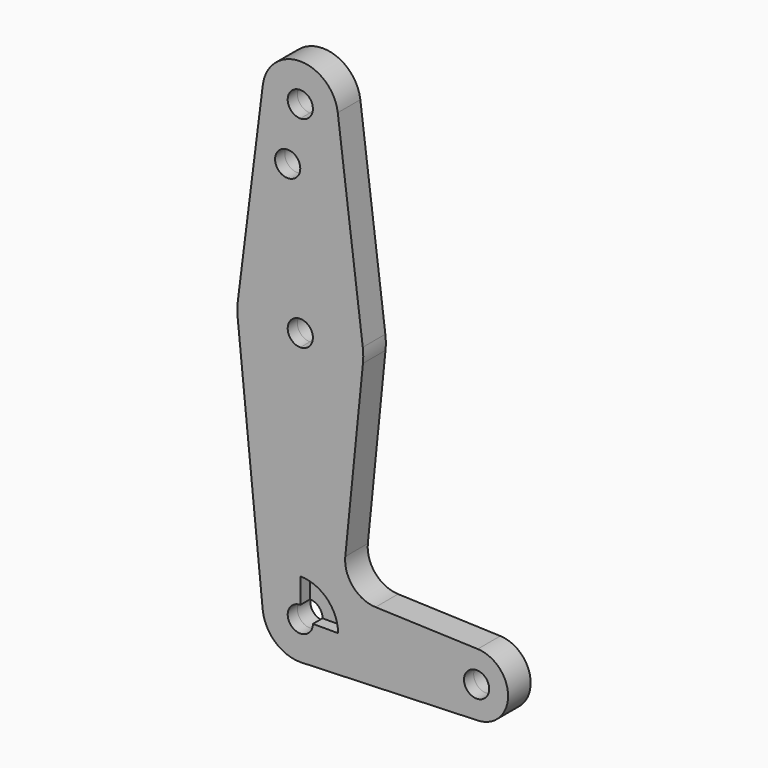
from build123d import *

# Parameters (mm, degrees)
F0_R     = 3.175
F1_DEPTH = 4.064
F2_DEPTH = 3.048


with BuildPart() as f1:
    # F0 (on Front) → F1 (new body)
    with BuildSketch(Plane.XZ):
        with BuildLine():
            ThreePointArc((15.7954255641, -1.5875), (15.8550939106, -0.7947465541), (15.875, 0))
            ThreePointArc((15.875, 0), (15.8438414904, 0.9941387366), (15.7504882737, 1.984375))
            ThreePointArc((15.7504882737, 1.984375), (10.5003255158, 11.90625), (0, 15.875))
            Line((0, 15.875), (0, 3.175))
            ThreePointArc((0, 3.175), (2.2450640303, 2.2450640303), (3.175, 0))
            ThreePointArc((3.175, 0), (2.2450640303, -2.2450640303), (0, -3.175))
            Line((0, -3.175), (0, -15.875))
            ThreePointArc((0, -15.875), (10.6492737428, -11.7732150983), (15.7954255641, -1.5875))
        make_face()
        with BuildLine():
            ThreePointArc((0, 15.875), (10.5003255158, 11.90625), (15.7504882737, 1.984375))
            Line((15.7504882737, 1.984375), (9.4502929642, 51.990625))
            ThreePointArc((9.4502929642, 51.990625), (9.5063048942, 51.396483242), (9.525, 50.8))
            ThreePointArc((9.525, 50.8), (6.7351920908, 44.0648079092), (0, 41.275))
            Line((0, 41.275), (0, 36.5252))
            Line((0, 36.5252), (0, 29.7381002456))
            Line((0, 29.7381002456), (0, 15.875))
        make_face()
        with BuildLine():
            Line((11.3411865923, -45.9066181876), (15.7954255641, -1.5875))
            ThreePointArc((15.7954255641, -1.5875), (10.6492737428, -11.7732150983), (0, -15.875))
            Line((0, -15.875), (0, -53.975))
            ThreePointArc((0, -53.975), (6.7351920908, -56.7648079092), (9.525, -63.5))
            Line((9.525, -63.5), (36.5125, -63.5))
            ThreePointArc((36.5125, -63.5), (38.9384772185, -57.7879930953), (44.7334821429, -55.5675637964))
            Line((44.7334821429, -55.5675637964), (18.9676000005, -54.6467662892))
            ThreePointArc((18.9676000005, -54.6467662892), (13.2611998974, -51.9286408502), (11.3411865923, -45.9066181876))
        make_face()
        with BuildLine():
            Line((0, 3.175), (0, 15.875))
            ThreePointArc((0, 15.875), (-10.5003255158, 11.90625), (-15.7504882737, 1.984375))
            ThreePointArc((-15.7504882737, 1.984375), (-15.8737438155, 0.1997054867), (-15.7954255641, -1.5875))
            ThreePointArc((-15.7954255641, -1.5875), (-10.6492737428, -11.7732150983), (0, -15.875))
            Line((0, -15.875), (0, -3.175))
            ThreePointArc((0, -3.175), (-3.175, 0), (0, 3.175))
        make_face()
        with BuildLine():
            ThreePointArc((-15.7504882737, 1.984375), (-10.5003255158, 11.90625), (0, 15.875))
            Line((0, 15.875), (0, 29.7381002456))
            Line((0, 29.7381002456), (0, 36.5252))
            Line((0, 36.5252), (0, 41.275))
            ThreePointArc((0, 41.275), (-7.14375, 44.4998046905), (-9.4502929642, 51.990625))
            Line((-9.4502929642, 51.990625), (-15.7504882737, 1.984375))
        make_face()
        with Locations((-3.175, 36.5252)):
            Circle(F0_R, mode=Mode.SUBTRACT)
        with BuildLine():
            ThreePointArc((9.525, 50.8), (9.5063048942, 51.396483242), (9.4502929642, 51.990625))
            ThreePointArc((9.4502929642, 51.990625), (0, 60.325), (-9.4502929642, 51.990625))
            ThreePointArc((-9.4502929642, 51.990625), (-7.14375, 44.4998046905), (0, 41.275))
            ThreePointArc((0, 41.275), (6.7351920908, 44.0648079092), (9.525, 50.8))
        make_face()
        with BuildLine():
            ThreePointArc((3.175, 50.8), (2.2450640303, 48.5549359697), (0, 47.625))
            ThreePointArc((0, 47.625), (-2.2450640303, 53.0450640303), (3.175, 50.8))
        make_face(mode=Mode.SUBTRACT)
        with BuildLine():
            Line((0, -53.975), (0, -15.875))
            ThreePointArc((0, -15.875), (-10.6492737428, -11.7732150983), (-15.7954255641, -1.5875))
            Line((-15.7954255641, -1.5875), (-9.4772553384, -64.4525))
            ThreePointArc((-9.4772553384, -64.4525), (-7.063929059, -57.1104357543), (0, -53.975))
        make_face()
        with BuildLine():
            Line((0, -60.325), (0, -53.975))
            ThreePointArc((0, -53.975), (-7.063929059, -57.1104357543), (-9.4772553384, -64.4525))
            ThreePointArc((-9.4772553384, -64.4525), (-6.3895642457, -70.563929059), (0, -73.025))
            Line((0, -73.025), (0.6773435479, -73.000885786))
            ThreePointArc((0.6773435479, -73.000885786), (6.9705567315, -69.9912990883), (9.525, -63.5))
            Line((9.525, -63.5), (3.175, -63.5))
            ThreePointArc((3.175, -63.5), (-2.2450640303, -65.7450640303), (0, -60.325))
        make_face()
        with BuildLine():
            Line((36.5125, -63.5), (9.525, -63.5))
            ThreePointArc((9.525, -63.5), (6.9705567315, -69.9912990883), (0.6773435479, -73.000885786))
            Line((0.6773435479, -73.000885786), (44.7324052746, -71.4324746146))
            ThreePointArc((44.7324052746, -71.4324746146), (38.9380895153, -69.2116327839), (36.5125, -63.5))
        make_face()
        with BuildLine():
            ThreePointArc((52.3875, -63.5), (50.1620069047, -57.9884772185), (44.7334821429, -55.5675637964))
            ThreePointArc((44.7334821429, -55.5675637964), (38.9384772185, -57.7879930953), (36.5125, -63.5))
            ThreePointArc((36.5125, -63.5), (38.9380895153, -69.2116327839), (44.7324052746, -71.4324746146))
            ThreePointArc((44.7324052746, -71.4324746146), (50.1616327839, -69.0119104847), (52.3875, -63.5))
        make_face()
        with BuildLine():
            ThreePointArc((47.625, -63.5), (44.45, -66.675), (41.275, -63.5))
            ThreePointArc((41.275, -63.5), (44.45, -60.325), (47.625, -63.5))
        make_face(mode=Mode.SUBTRACT)
        with BuildLine():
            Line((0.6773435479, -73.000885786), (0, -73.025))
            ThreePointArc((0, -73.025), (0.3388863295, -73.0189695375), (0.6773435479, -73.000885786))
        make_face()
        with BuildLine():
            ThreePointArc((9.525, -63.5), (6.7351920908, -56.7648079092), (0, -53.975))
            Line((0, -53.975), (0, -60.325))
            ThreePointArc((0, -60.325), (2.2450640303, -61.2549359697), (3.175, -63.5))
            Line((3.175, -63.5), (9.525, -63.5))
        make_face()
    extrude(amount=-F1_DEPTH)

    # F0 (on Front) → F2 (join)
    with BuildSketch(Plane.XZ):
        with BuildLine():
            ThreePointArc((15.7954255641, -1.5875), (15.8550939106, -0.7947465541), (15.875, 0))
            ThreePointArc((15.875, 0), (15.8438414904, 0.9941387366), (15.7504882737, 1.984375))
            ThreePointArc((15.7504882737, 1.984375), (10.5003255158, 11.90625), (0, 15.875))
            Line((0, 15.875), (0, 3.175))
            ThreePointArc((0, 3.175), (2.2450640303, 2.2450640303), (3.175, 0))
            ThreePointArc((3.175, 0), (2.2450640303, -2.2450640303), (0, -3.175))
            Line((0, -3.175), (0, -15.875))
            ThreePointArc((0, -15.875), (10.6492737428, -11.7732150983), (15.7954255641, -1.5875))
        make_face()
        with BuildLine():
            ThreePointArc((0, 15.875), (10.5003255158, 11.90625), (15.7504882737, 1.984375))
            Line((15.7504882737, 1.984375), (9.4502929642, 51.990625))
            ThreePointArc((9.4502929642, 51.990625), (9.5063048942, 51.396483242), (9.525, 50.8))
            ThreePointArc((9.525, 50.8), (6.7351920908, 44.0648079092), (0, 41.275))
            Line((0, 41.275), (0, 36.5252))
            Line((0, 36.5252), (0, 29.7381002456))
            Line((0, 29.7381002456), (0, 15.875))
        make_face()
        with BuildLine():
            Line((11.3411865923, -45.9066181876), (15.7954255641, -1.5875))
            ThreePointArc((15.7954255641, -1.5875), (10.6492737428, -11.7732150983), (0, -15.875))
            Line((0, -15.875), (0, -53.975))
            ThreePointArc((0, -53.975), (6.7351920908, -56.7648079092), (9.525, -63.5))
            Line((9.525, -63.5), (36.5125, -63.5))
            ThreePointArc((36.5125, -63.5), (38.9384772185, -57.7879930953), (44.7334821429, -55.5675637964))
            Line((44.7334821429, -55.5675637964), (18.9676000005, -54.6467662892))
            ThreePointArc((18.9676000005, -54.6467662892), (13.2611998974, -51.9286408502), (11.3411865923, -45.9066181876))
        make_face()
        with BuildLine():
            Line((0, 3.175), (0, 15.875))
            ThreePointArc((0, 15.875), (-10.5003255158, 11.90625), (-15.7504882737, 1.984375))
            ThreePointArc((-15.7504882737, 1.984375), (-15.8737438155, 0.1997054867), (-15.7954255641, -1.5875))
            ThreePointArc((-15.7954255641, -1.5875), (-10.6492737428, -11.7732150983), (0, -15.875))
            Line((0, -15.875), (0, -3.175))
            ThreePointArc((0, -3.175), (-3.175, 0), (0, 3.175))
        make_face()
        with BuildLine():
            ThreePointArc((-15.7504882737, 1.984375), (-10.5003255158, 11.90625), (0, 15.875))
            Line((0, 15.875), (0, 29.7381002456))
            Line((0, 29.7381002456), (0, 36.5252))
            Line((0, 36.5252), (0, 41.275))
            ThreePointArc((0, 41.275), (-7.14375, 44.4998046905), (-9.4502929642, 51.990625))
            Line((-9.4502929642, 51.990625), (-15.7504882737, 1.984375))
        make_face()
        with Locations((-3.175, 36.5252)):
            Circle(F0_R, mode=Mode.SUBTRACT)
        with BuildLine():
            ThreePointArc((9.525, 50.8), (9.5063048942, 51.396483242), (9.4502929642, 51.990625))
            ThreePointArc((9.4502929642, 51.990625), (0, 60.325), (-9.4502929642, 51.990625))
            ThreePointArc((-9.4502929642, 51.990625), (-7.14375, 44.4998046905), (0, 41.275))
            ThreePointArc((0, 41.275), (6.7351920908, 44.0648079092), (9.525, 50.8))
        make_face()
        with BuildLine():
            ThreePointArc((3.175, 50.8), (2.2450640303, 48.5549359697), (0, 47.625))
            ThreePointArc((0, 47.625), (-2.2450640303, 53.0450640303), (3.175, 50.8))
        make_face(mode=Mode.SUBTRACT)
        with BuildLine():
            Line((0, -53.975), (0, -15.875))
            ThreePointArc((0, -15.875), (-10.6492737428, -11.7732150983), (-15.7954255641, -1.5875))
            Line((-15.7954255641, -1.5875), (-9.4772553384, -64.4525))
            ThreePointArc((-9.4772553384, -64.4525), (-7.063929059, -57.1104357543), (0, -53.975))
        make_face()
        with BuildLine():
            Line((0, -60.325), (0, -53.975))
            ThreePointArc((0, -53.975), (-7.063929059, -57.1104357543), (-9.4772553384, -64.4525))
            ThreePointArc((-9.4772553384, -64.4525), (-6.3895642457, -70.563929059), (0, -73.025))
            Line((0, -73.025), (0.6773435479, -73.000885786))
            ThreePointArc((0.6773435479, -73.000885786), (6.9705567315, -69.9912990883), (9.525, -63.5))
            Line((9.525, -63.5), (3.175, -63.5))
            ThreePointArc((3.175, -63.5), (-2.2450640303, -65.7450640303), (0, -60.325))
        make_face()
        with BuildLine():
            Line((36.5125, -63.5), (9.525, -63.5))
            ThreePointArc((9.525, -63.5), (6.9705567315, -69.9912990883), (0.6773435479, -73.000885786))
            Line((0.6773435479, -73.000885786), (44.7324052746, -71.4324746146))
            ThreePointArc((44.7324052746, -71.4324746146), (38.9380895153, -69.2116327839), (36.5125, -63.5))
        make_face()
        with BuildLine():
            ThreePointArc((52.3875, -63.5), (50.1620069047, -57.9884772185), (44.7334821429, -55.5675637964))
            ThreePointArc((44.7334821429, -55.5675637964), (38.9384772185, -57.7879930953), (36.5125, -63.5))
            ThreePointArc((36.5125, -63.5), (38.9380895153, -69.2116327839), (44.7324052746, -71.4324746146))
            ThreePointArc((44.7324052746, -71.4324746146), (50.1616327839, -69.0119104847), (52.3875, -63.5))
        make_face()
        with BuildLine():
            ThreePointArc((47.625, -63.5), (44.45, -66.675), (41.275, -63.5))
            ThreePointArc((41.275, -63.5), (44.45, -60.325), (47.625, -63.5))
        make_face(mode=Mode.SUBTRACT)
        with BuildLine():
            Line((0.6773435479, -73.000885786), (0, -73.025))
            ThreePointArc((0, -73.025), (0.3388863295, -73.0189695375), (0.6773435479, -73.000885786))
        make_face()
    extrude(amount=F2_DEPTH)


solid = f1.part
